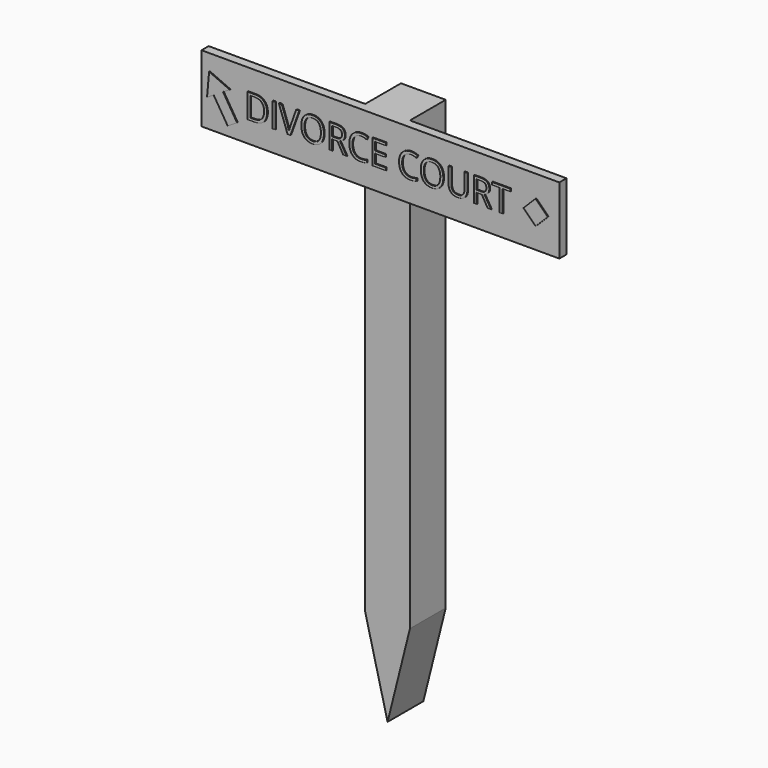
from build123d import *

# Parameters (mm, degrees)
F0_W         = 101.6
F0_H         = 19.05
F1_DEPTH     = 2.54
F2_TEXT_SIZE = 9.7551608257
F3_DEPTH     = 0.254
F4_W         = 12.7
F4_H         = 19.05
F5_DEPTH     = 12.7


# Not quite as in the source:
# - Text() gives the source's letters only with a copy of the font that has no kerning and outlines rounded to 1/6400 em; it was checked with that copy


with BuildPart() as f1:
    # F0 (on Front) → F1 (new body)
    with BuildSketch(Plane.XZ):
        Rectangle(F0_W, F0_H)
    extrude(amount=F1_DEPTH)

    # F2 (on face) → F3 (join)
    with BuildSketch(Plane.XZ.offset(2.54)):
        Polygon((44.2744009197, 3.4576579928), (40.8167429268, 0), (44.2744009197, -3.4576579928), (47.7320589125, 0), align=None)
        Polygon((-44.4840431065, 1.277224081), (-42.5993315876, 2.4439487606), (-48.4341345727, 5.0371945836), (-49.0271829379, -1.5351922018), (-47.142471419, -0.3684675222), (-43.1602605446, -6.8012779675), (-40.5018322321, -5.1555863643), align=None)
        with Locations((-38.4766208999, -3.374011975)):
            Text('DIVORCE COURT', F2_TEXT_SIZE, font='Open Sans', text_align=(TextAlign.LEFT, TextAlign.BOTTOM))
    extrude(amount=F3_DEPTH)

    # F4 (on face) → F5 (join)
    with BuildSketch(Plane(origin=(0, 0, 0), x_dir=(-1, 0, 0), z_dir=(0, 1, 0))):
        Rectangle(F4_W, F4_H)
        Polygon((6.35, -9.525), (-6.35, -9.525), (-6.35, -117.475), (0, -142.875), (6.35, -117.475), align=None)
    extrude(amount=F5_DEPTH)


solid = f1.part
